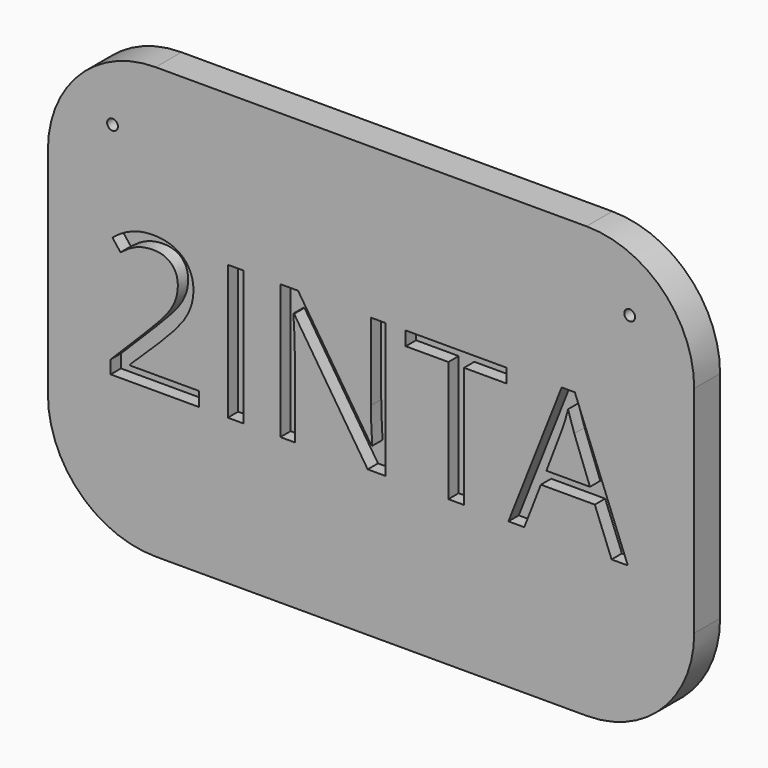
from build123d import *

# Parameters (mm, degrees)
F0_W         = 300
F0_H         = 200
F1_DEPTH     = 15
F3_R         = 50
F2_TEXT_SIZE = 87.5560906206
F4_DEPTH     = 6
F5_R         = 2.5
F6_DEPTH     = 25


# Not quite as in the source:
# - Text() gives the source's letters only with a copy of the font that has no kerning and outlines rounded to 1/6400 em; it was checked with that copy


with BuildPart() as f1:
    # F0 (on Front) → F1 (new body)
    with BuildSketch(Plane.XZ):
        Rectangle(F0_W, F0_H)
    extrude(amount=F1_DEPTH)

    # F3
    f3_edges = [f1.edges().sort_by_distance(p)[0] for p in [
        (150, -7.5, 100),
        (150, -7.5, -100),
        (-150, -7.5, -100),
        (-150, -7.5, 100),
    ]]
    fillet(f3_edges, radius=F3_R)

    # F2 (on face) → F4 (cut)
    with BuildSketch(Plane.XZ.offset(15)):
        with Locations((-125.1594365826, -32.3417070934)):
            Text('2INTA', F2_TEXT_SIZE, font='Open Sans', text_align=(TextAlign.LEFT, TextAlign.BOTTOM))
    extrude(amount=-F4_DEPTH, mode=Mode.SUBTRACT)

    # F5 (on face) → F6 (cut)
    with BuildSketch(Plane.XZ.offset(15)):
        with Locations((-120, 70)):
            Circle(F5_R)
        with Locations((120.0423410253, 70.1698749389)):
            Circle(F5_R)
    extrude(amount=-F6_DEPTH, mode=Mode.SUBTRACT)


solid = f1.part
